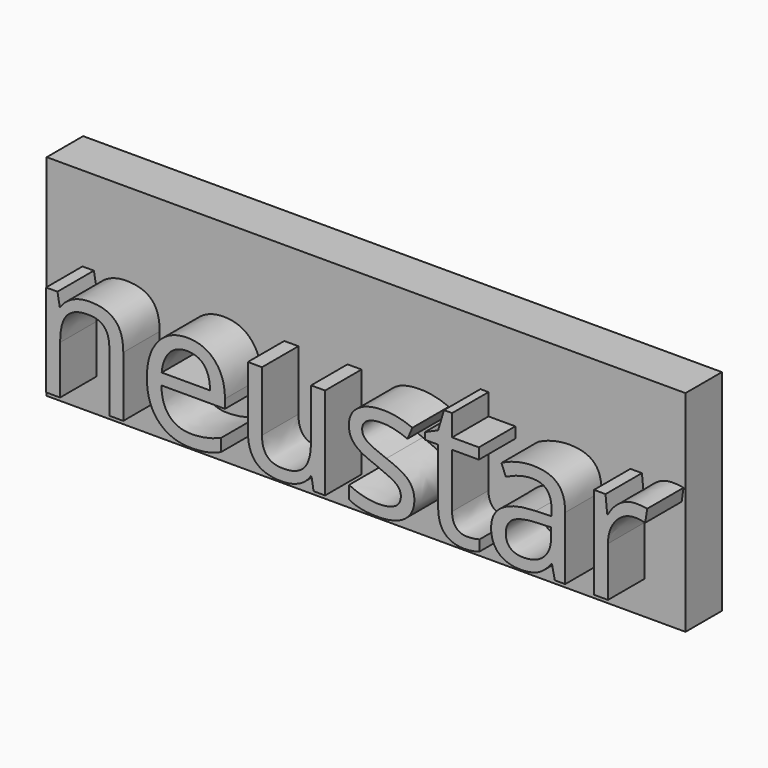
from build123d import *

# Parameters (mm, degrees)
F0_TEXT_SIZE = 48.1526470847
F1_DEPTH     = 12.7
F2_W         = 178.2208047807
F2_H         = 58.6427096277
F3_DEPTH     = 12.7


# Not quite as in the source:
# - Text() gives the source's letters only with a copy of the font that has no kerning and outlines rounded to 1/6400 em; it was checked with that copy


with BuildPart() as f1:
    # F0 (on Front) → F1 (new body)
    with BuildSketch(Plane.XZ):
        with Locations((-43.7140665017, -9.6874460578)):
            Text('neustar', F0_TEXT_SIZE, font='Open Sans', text_align=(TextAlign.LEFT, TextAlign.BOTTOM))
    extrude(amount=F1_DEPTH)


with BuildPart() as f3:
    # F2 (on Front) → F3 (new body)
    with BuildSketch(Plane.XZ):
        with Locations((39.5561922342, 10.3577440605)):
            Rectangle(F2_W, F2_H)
    extrude(amount=-F3_DEPTH)


solid = Compound([f1.part, f3.part])
